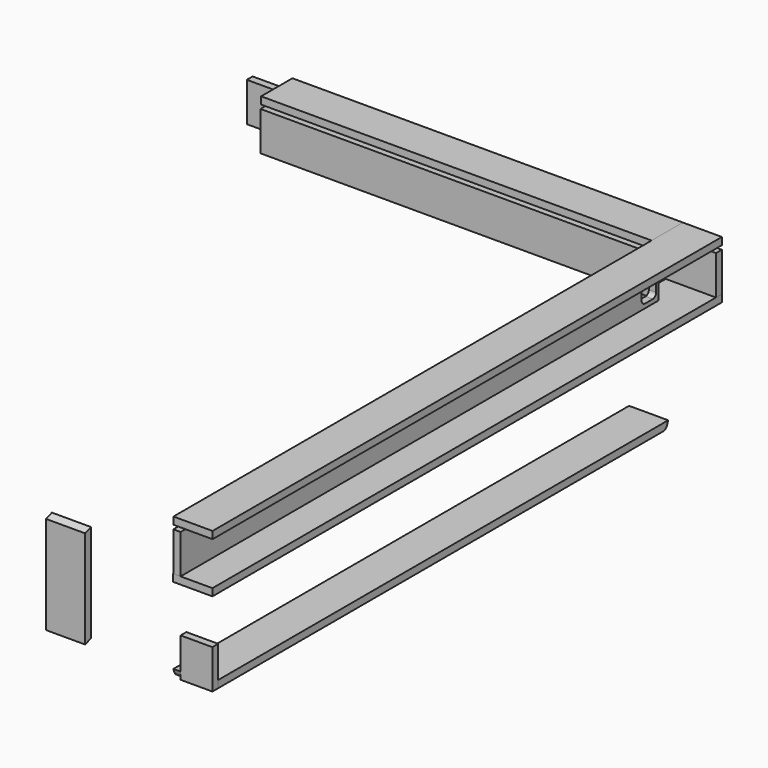
from build123d import *

# Parameters (mm, degrees)
F0_W        = 140
F0_H        = 26
F1_DEPTH    = 2040
F2_SIZE2    = 9.463216
F2_SIZE     = 25.99999
F2_2_SIZE2  = 9.463216
F2_2_SIZE   = 25.99999
F3_W        = 180
F3_H        = 26
F4_DEPTH    = 2280
F5_W        = 40
F5_H        = 140
F6_DEPTH    = 26
F7_W        = 114
F7_H        = 26
F8_DEPTH    = 140
F9_W        = 26
F9_H        = 140
F10_DEPTH   = 2140
F12_W       = 26
F12_H       = 140
F13_DEPTH   = 840
F14_W       = 26
F14_H       = 140
F15_DEPTH   = 700
F16_W       = 140
F16_H       = 26
F17_DEPTH   = 360
F18_SIZE2   = 9.463216
F18_SIZE    = 25.99999
F18_2_SIZE2 = 9.463216
F18_2_SIZE  = 25.99999
F19_W       = 140
F19_H       = 26
F20_DEPTH   = 700
F21_W       = 140
F21_H       = 26
F22_DEPTH   = 2280
F23_DEPTH   = 1566.001
F24_R       = 20


# Not quite as in the source:
# - a fillet or chamfer is up to 0.001 mm smaller than in the source, because OpenCascade refuses the exact size


with BuildPart() as f1:
    # F0 (on Front) → F1 (new body)
    with BuildSketch(Plane.XZ):
        with Locations((770, 13)):
            Rectangle(F0_W, F0_H)
    extrude(amount=-F1_DEPTH)

    # F2 (size 26 and 9.4632260909 in the source; OpenCascade refuses exactly that, so slightly less here)
    f2_edges = [f1.edges().sort_by_distance(p)[0] for p in [
        (770, 0, 0),
    ]]
    f2_side = f1.faces().sort_by_distance((770, 0, 13))[0]
    chamfer(f2_edges, length=F2_SIZE, length2=F2_SIZE2, reference=f2_side)

    # F2#2 (size 26 and 9.4632260909 in the source; OpenCascade refuses exactly that, so slightly less here)
    f2_2_edges = [f1.edges().sort_by_distance(p)[0] for p in [
        (770, 2040, 0),
    ]]
    f2_2_side = f1.faces().sort_by_distance((770, 2040, 13))[0]
    chamfer(f2_2_edges, length=F2_2_SIZE, length2=F2_2_SIZE2, reference=f2_2_side)

    # F24
    f24_edges = [f1.edges().sort_by_distance(p)[0] for p in [
        (770, 9.463216, 0),
        (770, 2030.536784, 0),
    ]]
    fillet(f24_edges, radius=F24_R)


with BuildPart() as f4:
    # F3 (on Front) → F4 (new body)
    with BuildSketch(Plane.XZ):
        with Locations((750, 313)):
            Rectangle(F3_W, F3_H)
    extrude(amount=-F4_DEPTH)

    # F5 (on face) → F6 (cut, through all)
    with BuildSketch(Plane.XY.offset(326)):
        with Locations((679.6356630325, 70)):
            Rectangle(F5_W, F5_H)
    extrude(amount=-F6_DEPTH, mode=Mode.SUBTRACT)


with BuildPart() as f8:
    # F7 (on Top) → F8 (new body)
    with BuildSketch(Plane.XY):
        with Locations((783, 13)):
            Rectangle(F7_W, F7_H)
    extrude(amount=F8_DEPTH)


with BuildPart() as f10:
    # F9 (on Front) → F10 (new body)
    with BuildSketch(Plane.XZ):
        with Locations((713, 396)):
            Rectangle(F9_W, F9_H)
    extrude(amount=-F10_DEPTH)

    # F11 (on face) → F23 (cut, through all)
    with BuildSketch(Plane.YZ.offset(726)):
        with BuildLine():
            ThreePointArc((2128.5, 436), (2124.1066017178, 446.6066017178), (2113.5, 451))
            Line((2113.5, 451), (2078.5, 451))
            ThreePointArc((2078.5, 451), (2067.8933982822, 446.6066017178), (2063.5, 436))
            Line((2063.5, 436), (2063.5, 356))
            ThreePointArc((2063.5, 356), (2067.8933982822, 345.3933982822), (2078.5, 341))
            Line((2078.5, 341), (2113.5, 341))
            ThreePointArc((2113.5, 341), (2124.1066017178, 345.3933982822), (2128.5, 356))
            Line((2128.5, 356), (2128.5, 436))
        make_face()
    extrude(amount=-F23_DEPTH, mode=Mode.SUBTRACT)


with BuildPart() as f13:
    # F12 (on Right) → F13 (new body, symmetric)
    with BuildSketch(Plane.YZ):
        with Locations((2267, 396)):
            Rectangle(F12_W, F12_H)
    extrude(amount=F13_DEPTH, both=True)


with BuildPart() as f15:
    # F14 (on Right) → F15 (new body, symmetric)
    with BuildSketch(Plane.YZ):
        with Locations((2153, 396)):
            Rectangle(F14_W, F14_H)
    extrude(amount=F15_DEPTH, both=True)


with BuildPart() as f17:
    # F16 (on Top) → F17 (new body)
    with BuildSketch(Plane.XY):
        with Locations((314.363963604, 13)):
            Rectangle(F16_W, F16_H)
    extrude(amount=F17_DEPTH)

    # F18 (size 26 and 9.4632260909 in the source; OpenCascade refuses exactly that, so slightly less here)
    f18_edges = [f17.edges().sort_by_distance(p)[0] for p in [
        (314.363964, 0, 360),
    ]]
    f18_side = f17.faces().sort_by_distance((314.363964, 13, 360))[0]
    chamfer(f18_edges, length=F18_SIZE, length2=F18_SIZE2, reference=f18_side)

    # F18#2 (size 26 and 9.4632260909 in the source; OpenCascade refuses exactly that, so slightly less here)
    f18_2_edges = [f17.edges().sort_by_distance(p)[0] for p in [
        (314.363964, 26, 0),
    ]]
    f18_2_side = f17.faces().sort_by_distance((314.363964, 13, 0))[0]
    chamfer(f18_2_edges, length=F18_2_SIZE, length2=F18_2_SIZE2, reference=f18_2_side)


with BuildPart() as f20:
    # F19 (on Right) → F20 (new body, symmetric)
    with BuildSketch(Plane.YZ):
        with Locations((2213.114566803, 491.5019755363)):
            Rectangle(F19_W, F19_H)
    extrude(amount=F20_DEPTH, both=True)


with BuildPart() as f22:
    # F21 (on Front) → F22 (new body)
    with BuildSketch(Plane.XZ):
        with Locations((770.4404592514, 493.4790836821)):
            Rectangle(F21_W, F21_H)
    extrude(amount=-F22_DEPTH)


solid = Compound([f1.part, f4.part, f8.part, f10.part, f13.part, f15.part, f17.part, f20.part, f22.part])
